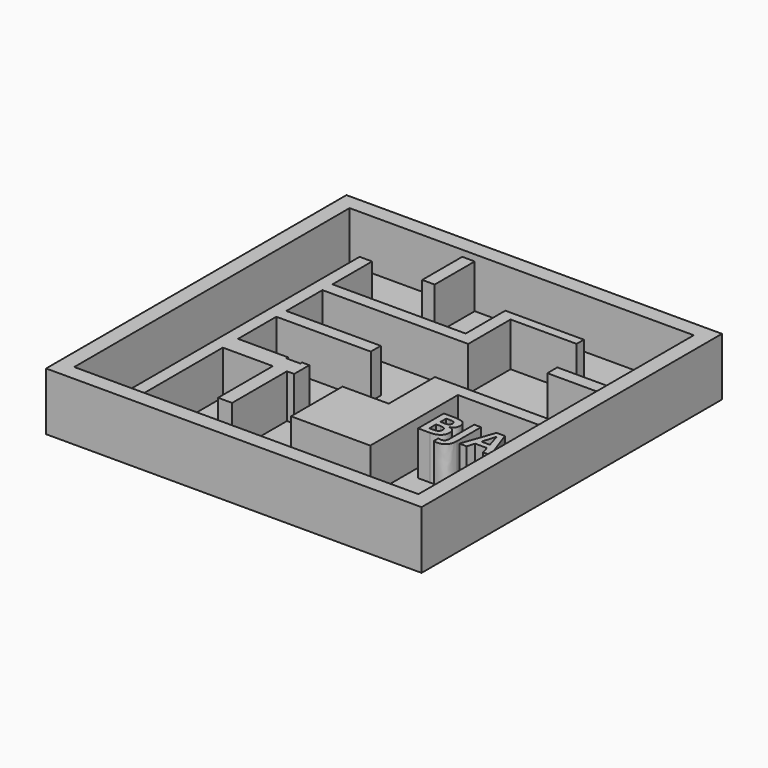
from build123d import *

# Parameters (mm, degrees)
F0_W         = 38.1
F0_H         = 38.1
F1_DEPTH     = 0.79375
F2_W         = 38.1
F2_H         = 38.1
F2_W_2       = 34.925
F2_H_2       = 34.925
F3_DEPTH     = 5.08
F4_R         = 1.27
F5_DEPTH     = 0.396875
F4_W         = 1.27
F4_H         = 5.08
F4_W_2       = 9.5824494671
F4_H_2       = 1.27
F4_W_3       = 5.7560304195
F4_TEXT_SIZE = 4.5861111111
F6_DEPTH     = 4.445


# Not quite as in the source:
# - Text() gives the source's letters only with a copy of the font that has no kerning and outlines rounded to 1/6400 em; it was checked with that copy


with BuildPart() as f1:
    # F0 (on Top) → F1 (new body)
    with BuildSketch(Plane.XY):
        with Locations((-0.5224868655, -6.0101259537)):
            Rectangle(F0_W, F0_H)
    extrude(amount=F1_DEPTH)

    # F2 (on face) → F3 (join)
    with BuildSketch(Plane.XY.offset(0.79375)):
        with Locations((-0.5224868655, -6.0101259537)):
            Rectangle(F2_W, F2_H)
        with Locations((-0.5224868655, -6.0101259537)):
            Rectangle(F2_W_2, F2_H_2, mode=Mode.SUBTRACT)
    extrude(amount=F3_DEPTH)

    # F4 (on face) → F5 (cut)
    with BuildSketch(Plane.XY.offset(0.79375)):
        with Locations((-15.4449868655, -19.2887317389)):
            Circle(F4_R)
        with Locations((7.8901294619, -21.2152693421)):
            Circle(F4_R)
    extrude(amount=-F5_DEPTH, mode=Mode.SUBTRACT)

    # F4 (on face) → F6 (join)
    with BuildSketch(Plane.XY.offset(0.79375)):
        Polygon((-12.9049868655, 6.3723740463), (-12.9049868655, -23.4726259537), (-11.6349868655, -23.4726259537), (-11.6349868655, -12.5638665631), (-11.6349868655, -10.6370309368), (-11.6349868655, -5.7780551724), (-11.6349868655, -4.5080551724), (-11.6349868655, 0.0728578386), (-11.6349868655, 1.3428578386), (-11.6349868655, 6.3723740463), align=None)
        with Locations((-5.9199868655, 8.9123740463)):
            Rectangle(F4_W, F4_H)
        Polygon((-6.5549868655, 1.3428578386), (-11.6349868655, 1.3428578386), (-11.6349868655, 0.0728578386), (3.154908881, 0.0728578386), (3.154908881, 1.3428578386), (3.154908881, 5.4478542879), (9.8569440809, 5.4478542879), (9.8569440809, 6.3723740463), (3.154908881, 6.3723740463), (1.884908881, 6.3723740463), (1.884908881, 1.3428578386), (-5.2849868655, 1.3428578386), align=None)
        with Locations((-6.843762132, -5.1430551724)):
            Rectangle(F4_W_2, F4_H_2)
        Polygon((-11.6349868655, -10.6370309368), (-11.6349868655, -12.5638665631), (-6.5549868655, -12.5638665631), (-6.5549868655, -19.5172280073), (-5.1308041935, -19.5172280073), (-5.1308041935, -12.5638665631), (-4.398250021, -12.5638665631), (-4.398250021, -10.6370309368), (-5.1308041935, -10.6370309368), (-5.1308041935, -10.8580551724), (-6.5549868655, -10.8580551724), (-6.5549868655, -10.6370309368), align=None)
        with Locations((14.0619979247, 0.7078578386)):
            Rectangle(F4_W_3, F4_H_2)
        Polygon((7.991639001, -7.2801259537), (16.9400131345, -7.2801259537), (16.9400131345, -6.0101259537), (4.6406211682, -6.0101259537), (4.6406211682, -7.2801259537), (4.6406211682, -8.5071239059), (4.6406211682, -11.8633601497), (-0.0508041935, -11.8633601497), (-0.0508041935, -18.3926259537), (4.6406211682, -18.3926259537), (7.991639001, -18.3926259537), align=None)
        with Locations((8.685878478, -13.7226533845)):
            Text('BJA', F4_TEXT_SIZE, font='Open Sans', font_style=FontStyle.BOLD, text_align=(TextAlign.LEFT, TextAlign.BOTTOM))
    extrude(amount=F6_DEPTH)


solid = f1.part
